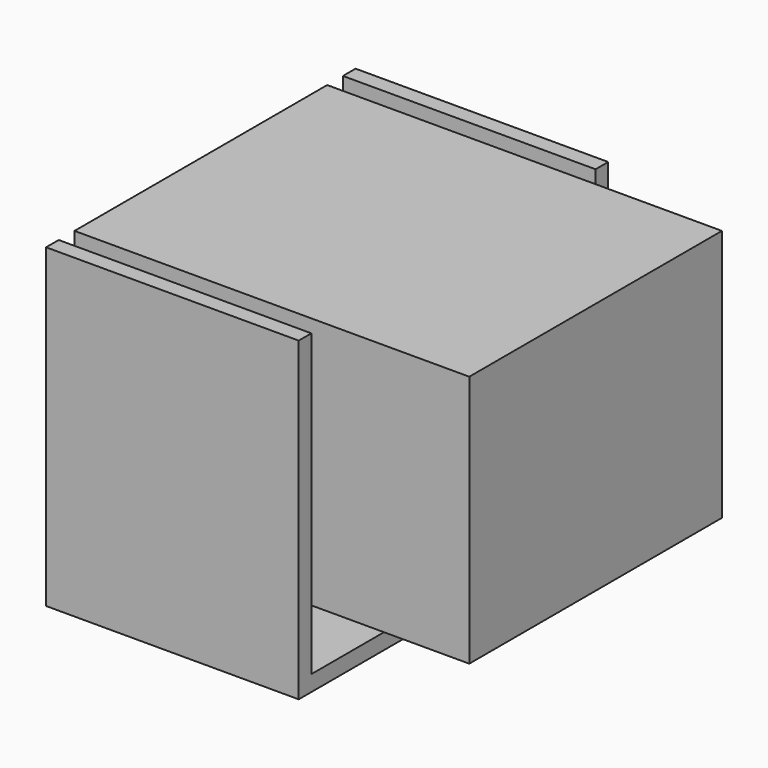
from build123d import *

# Parameters (mm, degrees)
F0_W     = 50
F0_H     = 32
F1_DEPTH = 40
F2_R     = 14
F3_DEPTH = 2
F4_R     = 14
F5_DEPTH = 2
F7_DEPTH = 32
F8_R     = 1.5
F9_DEPTH = 25


with BuildPart() as f1:
    # F0 (on Front) → F1 (new body)
    with BuildSketch(Plane.XZ):
        Rectangle(F0_W, F0_H)
    extrude(amount=F1_DEPTH)

    # F2 (on face) → F3 (join)
    with BuildSketch(Plane.XZ.offset(40)):
        with Locations((-9, 0)):
            Circle(F2_R)
    extrude(amount=F3_DEPTH)

    # F4 (on face) → F5 (join)
    with BuildSketch(Plane(origin=(0, 0, 0), x_dir=(-1, 0, 0), z_dir=(0, 1, 0))):
        with Locations((9, 0)):
            Circle(F4_R)
    extrude(amount=F5_DEPTH)


with BuildPart() as f7:
    # F6 (on face) → F7 (new body)
    with BuildSketch(Plane(origin=(-25, 0, 0), x_dir=(0, -1, 0), z_dir=(-1, 0, 0))):
        Polygon((-2.5, -22), (-2.5, 16), (-4.5, 16), (-4.5, -24), (44.5, -24), (44.5, 16), (42.5, 16), (42.5, -22), align=None)
    extrude(amount=-F7_DEPTH)

    # F8 (on face) → F9 (cut)
    with BuildSketch(Plane(origin=(0, 0, -24), x_dir=(1, 0, 0), z_dir=(0, 0, -1))):
        with Locations((-9, 20)):
            Circle(F8_R)
    extrude(amount=-F9_DEPTH, mode=Mode.SUBTRACT)


solid = Compound([f1.part, f7.part])
